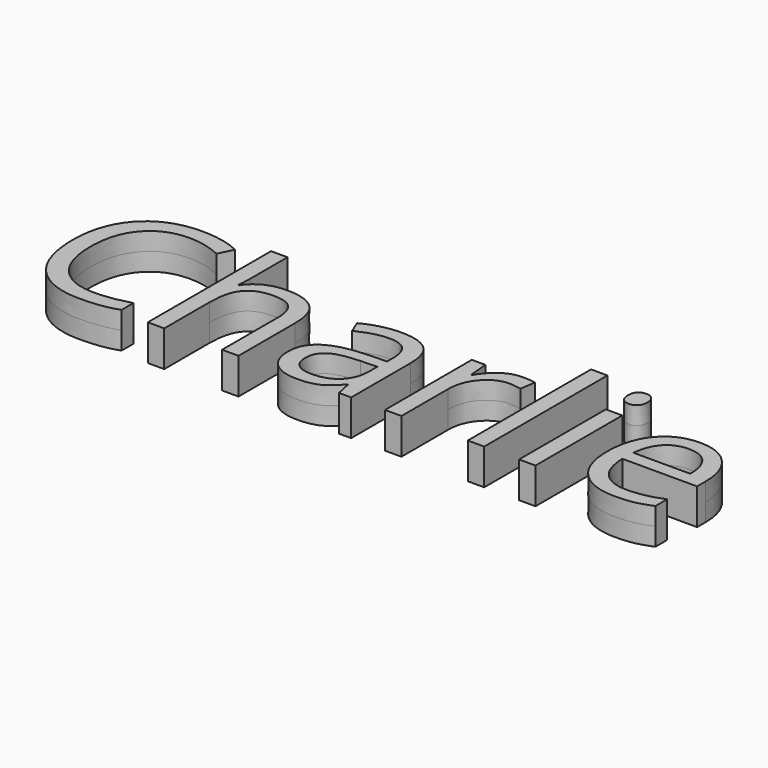
from build123d import *

# Parameters (mm, degrees)
F0_TEXT_SIZE = 71.7790771483
F1_DEPTH     = 6.35


# Not quite as in the source:
# - Text() gives the source's letters only with a copy of the font that has no kerning and outlines rounded to 1/6400 em; it was checked with that copy


with BuildPart() as f1:
    # F0 (on Top) → F1 (new body, symmetric)
    with BuildSketch(Plane.XY):
        with Locations((-116.4416223764, -22.65028283)):
            Text('Charlie', F0_TEXT_SIZE, font='Open Sans', text_align=(TextAlign.LEFT, TextAlign.BOTTOM))
    extrude(amount=F1_DEPTH, both=True)


solid = f1.part
